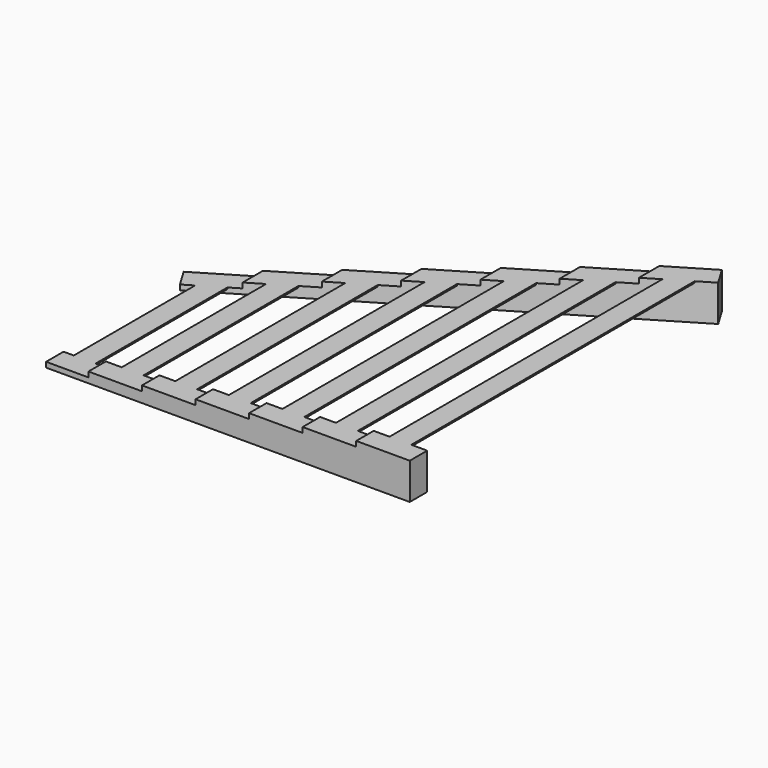
from build123d import *

# Parameters (mm, degrees)
F0_W     = 50
F0_H     = 3
F1_DEPTH = 5
F3_DEPTH = 55.5734787771
F4_W     = 3
F4_H     = 0.2
F5_REACH = 58.5801380528


with BuildPart() as f1:
    # F0 (on Top) → F1 (new body)
    with BuildSketch(Plane.XY):
        Rectangle(F0_W, F0_H)
    extrude(amount=F1_DEPTH)


with BuildPart() as f1b:
    # F0 (on Top) → F1, piece 2 (new body)
    with BuildSketch(Plane.XY):
        Polygon((-26.5434872663, 24.0724787771), (-25, 21.5), (25, 51.5), (23.4565127337, 54.0724787771), align=None)
    extrude(amount=F1_DEPTH)


with BuildPart() as f3_tool:
    # F2 (on face) → F3 (new body, through all)
    with BuildSketch(Plane.XZ.offset(1.5)):
        Polygon((17.6366446762, 5), (-26.5434872663, 5), (-26.5434872663, 0.7142857143), (-19.1801319425, 0.7142857143), (-19.1801319425, 1.4285714286), (-11.8167766188, 1.4285714286), (-11.8167766188, 2.1428571429), (-4.453421295, 2.1428571429), (-4.453421295, 2.8571428571), (2.9099340287, 2.8571428571), (2.9099340287, 3.5714285714), (10.2732893525, 3.5714285714), (10.2732893525, 4.2857142857), (17.6366446762, 4.2857142857), align=None)
    extrude(amount=-F3_DEPTH)


with BuildPart() as f1_1:
    add(f1.part)

    # F3: cut by f3_tool
    add(f3_tool.part, mode=Mode.SUBTRACT)



with BuildPart() as f1b_1:
    add(f1b.part)

    # F3: cut by f3_tool
    add(f3_tool.part, mode=Mode.SUBTRACT)


with BuildPart() as f1_2:
    add(f1_1.part)

    add(f1b_1.part)  # F5 merges F1b
    f5_end = f1_2.faces().sort_by_distance((5.616262324, 43.3683285313, 1.7462125476))[0]
    # F4 (on face) → F5 (join, up to a face of the model that its end follows)
    with BuildSketch(Plane.XZ.offset(1.5)):
        with Locations((-22.0900659713, 0.6142857143)):
            Rectangle(F4_W, F4_H)
        with Locations((-15.4984542807, 1.3285714286)):
            Rectangle(F4_W, F4_H)
        with Locations((-8.1350989569, 2.0428571429)):
            Rectangle(F4_W, F4_H)
        with Locations((-0.7717436331, 2.7571428571)):
            Rectangle(F4_W, F4_H)
        with Locations((6.5916116906, 3.4714285714)):
            Rectangle(F4_W, F4_H)
        with Locations((13.9549670144, 4.1857142857)):
            Rectangle(F4_W, F4_H)
        with Locations((21.3183223381, 4.9)):
            Rectangle(F4_W, F4_H)
    f5_long = extrude(amount=-F5_REACH, mode=Mode.PRIVATE)
    add(split(f5_long, bisect_by=f5_end, keep=Keep.BOTTOM, mode=Mode.PRIVATE))


solid = f1_2.part
